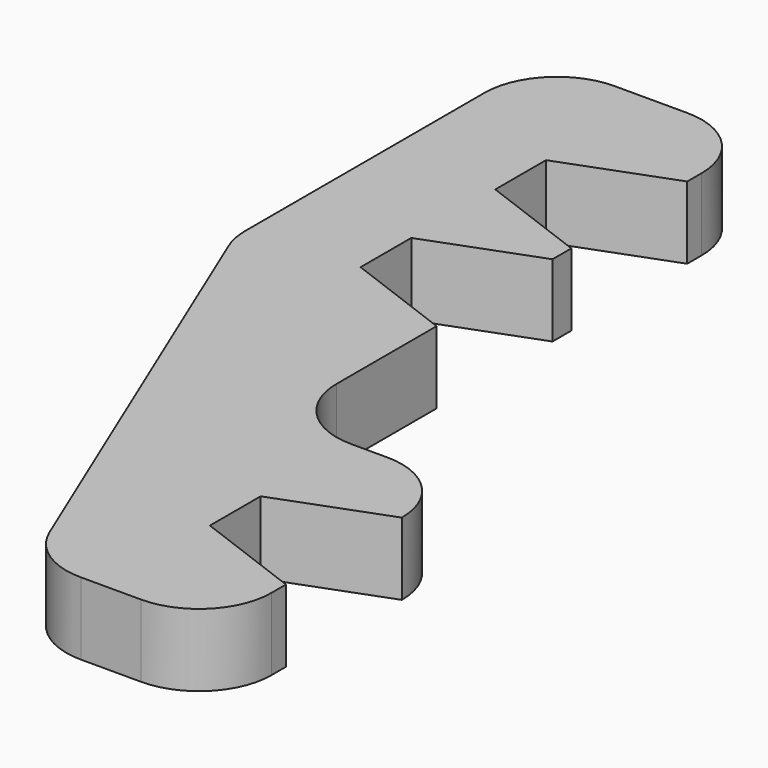
from build123d import *

# Parameters (mm, degrees)
F1_DEPTH     = 2
F2_R         = 2
F3_R         = 2
F4_T4_DEPTH  = 22.7509646446
F4_T9_DEPTH  = 22.7509646446
F4_T14_DEPTH = 22.7509646446
F5_T4_DEPTH  = 22.7509646446
F5_T9_DEPTH  = 22.7509646446
F6_T4_DEPTH  = 22.7509646446


# Not quite as in the source:
# - a fillet or chamfer that OpenCascade refuses, or shapes differently, is made with other operations: its cross-section is extruded or revolved along the edge and cut away or added


with BuildPart() as f1:
    # F0 (on Top) → F1 (new body)
    with BuildSketch(Plane.XY):
        Polygon((-8.2, 10.65), (-14.2, 10.65), (-14.2, 0), (-8.2, -14.45), (-3.2, -14.45), (-3.2, -10.45), (-6.2, -10.45), (-6.2, -9.45), (-3.2, -9.45), (-3.2, -5.95), (-8.2, -5.95), (-8.2, 1), (-11.2, 1), (-11.2, 2), (-8.2, 2), (-8.2, 5.65), (-11.2, 5.65), (-11.2, 6.65), (-8.2, 6.65), align=None)
    extrude(amount=F1_DEPTH)

    # F2
    f2_edges = [f1.edges().sort_by_distance(p)[0] for p in [
        (-14.2, 10.65, 1),
        (-14.2, 0, 1),
        (-8.2, 10.65, 1),
        (-8.2, -14.45, 1),
        (-3.2, -14.45, 1),
        (-3.2, -5.95, 1),
    ]]
    fillet(f2_edges, radius=F2_R)

    # F3
    f3_edges = [f1.edges().sort_by_distance(p)[0] for p in [
        (-8.2, -5.95, 1),
    ]]
    fillet(f3_edges, radius=F3_R)

    # F4: chamfer of 1.5 x 4 on 3 edges, made by hand


with BuildPart() as f4_tool2:
    # F4_s3 → F4_t4 (new body)
    with BuildSketch(Plane.XY.offset(-10.3754823223)):
        Polygon((-12.2, 6.65), (-8.2, 8.15), (-8.2, 6.65), align=None)
    extrude(amount=F4_T4_DEPTH)

    split(bisect_by=Plane.YZ.offset(-11.2), keep=Keep.TOP)


with BuildPart() as f1_1:
    add(f1.part)

    # F4_t1: cut F4_tool2
    add(f4_tool2.part, mode=Mode.SUBTRACT)


with BuildPart() as f4_tool7:
    # F4_s8 → F4_t9 (new body)
    with BuildSketch(Plane.XY.offset(-10.3754823223)):
        Polygon((-12.2, 2), (-8.2, 3.5), (-8.2, 2), align=None)
    extrude(amount=F4_T9_DEPTH)

    split(bisect_by=Plane.YZ.offset(-11.2), keep=Keep.TOP)


with BuildPart() as f1_2:
    add(f1_1.part)

    # F4_t6: cut F4_tool7
    add(f4_tool7.part, mode=Mode.SUBTRACT)


with BuildPart() as f4_tool12:
    # F4_s13 → F4_t14 (new body)
    with BuildSketch(Plane.XY.offset(-10.3754823223)):
        Polygon((-3.2, -7.95), (-7.2, -9.45), (-3.2, -9.45), align=None)
    extrude(amount=F4_T14_DEPTH)

    split(bisect_by=Plane.YZ.offset(-6.2), keep=Keep.TOP)


with BuildPart() as f1_3:
    add(f1_2.part)

    # F4_t11: cut F4_tool12
    add(f4_tool12.part, mode=Mode.SUBTRACT)

    # F5: chamfer of 4 x 1.5 on 2 edges, made by hand


with BuildPart() as f5_tool2:
    # F5_s3 → F5_t4 (new body)
    with BuildSketch(Plane.XY.offset(-10.3754823223)):
        Polygon((-12.2, 5.65), (-8.2, 4.15), (-8.2, 5.65), align=None)
    extrude(amount=F5_T4_DEPTH)

    split(bisect_by=Plane.YZ.offset(-11.2), keep=Keep.TOP)


with BuildPart() as f1_4:
    add(f1_3.part)

    # F5_t1: cut F5_tool2
    add(f5_tool2.part, mode=Mode.SUBTRACT)


with BuildPart() as f5_tool7:
    # F5_s8 → F5_t9 (new body)
    with BuildSketch(Plane.XY.offset(-10.3754823223)):
        Polygon((-7.2, -10.45), (-3.2, -11.95), (-3.2, -10.45), align=None)
    extrude(amount=F5_T9_DEPTH)

    split(bisect_by=Plane.YZ.offset(-6.2), keep=Keep.TOP)


with BuildPart() as f1_5:
    add(f1_4.part)

    # F5_t6: cut F5_tool7
    add(f5_tool7.part, mode=Mode.SUBTRACT)

    # F6: chamfer of 4 x 1.5 on 1 edges, made by hand


with BuildPart() as f6_tool2:
    # F6_s3 → F6_t4 (new body)
    with BuildSketch(Plane.XY.offset(-10.3754823223)):
        Polygon((-12.2, 1), (-8.2, -0.5), (-8.2, 1), align=None)
    extrude(amount=F6_T4_DEPTH)

    split(bisect_by=Plane.YZ.offset(-11.2), keep=Keep.TOP)


with BuildPart() as f1_6:
    add(f1_5.part)

    # F6_t1: cut F6_tool2
    add(f6_tool2.part, mode=Mode.SUBTRACT)


solid = f1_6.part
